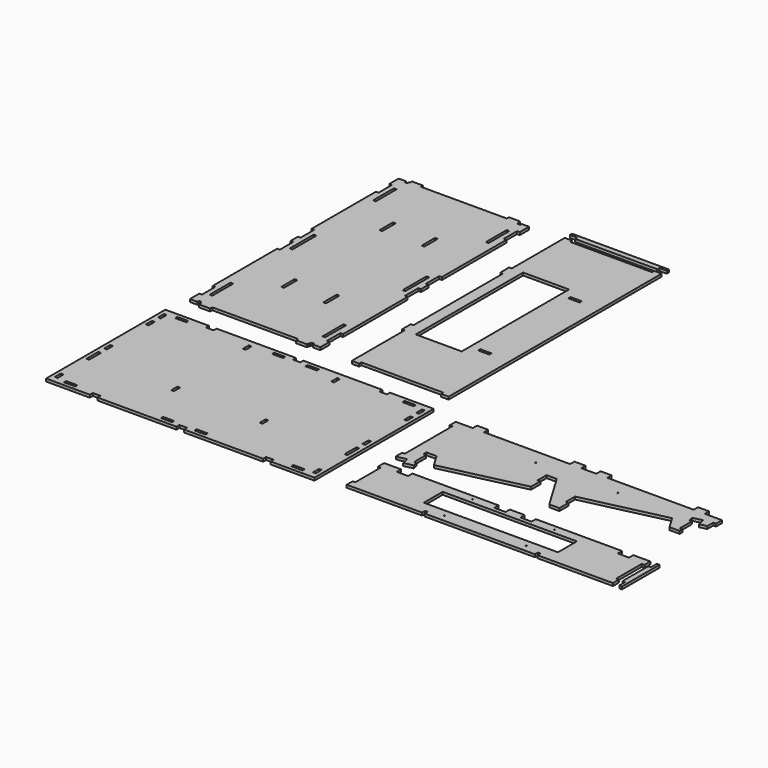
from build123d import *

# Parameters (mm, degrees)
F1_W     = 18.288
F1_H     = 177.8
F1_H_2   = 114.3
F1_H_3   = 203.2
F1_W_2   = 76.2
F1_H_4   = 18.288
F2_DEPTH = 18.288
F1_W_3   = 50.8
F1_H_5   = 76.2
F1_W_4   = 558.8
F1_H_6   = 50.8
F1_R     = 3.4925
F1_H_7   = 36.576
F1_H_8   = 25.4
F1_W_5   = 914.4
F1_H_9   = 161.1005576621
F1_H_10  = 217.424


# Not quite as in the source:
# - a variable given as a bare number and used for a length is read in inches; the dataset says mm whatever the document's units were


with BuildPart() as f2:
    # F1 (on Top) → F2 (new body)
    with BuildSketch(Plane.XY):
        Polygon((-889, 764.9814906911), (-889, 685.8), (-838.2, 685.8), (-838.2, 698.5), (-819.912, 698.5), (-819.912, 685.8), (-812.8, 685.8), (-736.6, 685.8), (-152.4, 685.8), (-76.2, 685.8), (-69.088, 685.8), (-69.088, 698.5), (-50.8, 698.5), (-50.8, 685.8), (0, 685.8), (0, 764.9814906911), (-18.288, 764.9814906911), (-18.288, 879.2814906911), (0, 879.2814906911), (0, 1428.75), (-18.288, 1428.75), (-18.288, 1543.05), (0, 1543.05), (0, 1606.55), (-18.288, 1606.55), (-18.288, 1720.85), (0, 1720.85), (0, 2270.3185093089), (-18.288, 2270.3185093089), (-18.288, 2384.6185093089), (0, 2384.6185093089), (0, 2463.8), (-50.8, 2463.8), (-50.8, 2451.1), (-69.088, 2451.1), (-69.088, 2463.8), (-76.2, 2463.8), (-152.4, 2463.8), (-736.6, 2463.8), (-812.8, 2463.8), (-819.912, 2463.8), (-819.912, 2451.1), (-838.2, 2451.1), (-838.2, 2463.8), (-889, 2463.8), (-889, 2384.6185093089), (-870.712, 2384.6185093089), (-870.712, 2270.3185093089), (-889, 2270.3185093089), (-889, 1720.85), (-870.712, 1720.85), (-870.712, 1606.55), (-889, 1606.55), (-889, 1543.05), (-870.712, 1543.05), (-870.712, 1428.75), (-889, 1428.75), (-889, 879.2814906911), (-870.712, 879.2814906911), (-870.712, 764.9814906911), align=None)
        with Locations((-829.056, 878.8908)):
            Rectangle(F1_W, F1_H, mode=Mode.SUBTRACT)
        with Locations((-59.944, 878.8908)):
            Rectangle(F1_W, F1_H, mode=Mode.SUBTRACT)
        with Locations((-587.756, 1155.7)):
            Rectangle(F1_W, F1_H_2, mode=Mode.SUBTRACT)
        with Locations((-301.244, 1155.7)):
            Rectangle(F1_W, F1_H_2, mode=Mode.SUBTRACT)
        with Locations((-829.056, 1574.8)):
            Rectangle(F1_W, F1_H_3, mode=Mode.SUBTRACT)
        with Locations((-59.944, 1574.8)):
            Rectangle(F1_W, F1_H_3, mode=Mode.SUBTRACT)
        with Locations((-587.756, 1993.9)):
            Rectangle(F1_W, F1_H_2, mode=Mode.SUBTRACT)
        with Locations((-301.244, 1993.9)):
            Rectangle(F1_W, F1_H_2, mode=Mode.SUBTRACT)
        with Locations((-829.056, 2270.7092)):
            Rectangle(F1_W, F1_H, mode=Mode.SUBTRACT)
        with Locations((-59.944, 2270.7092)):
            Rectangle(F1_W, F1_H, mode=Mode.SUBTRACT)
        with Locations((-774.7, 2472.944)):
            Rectangle(F1_W_2, F1_H_4)
        with Locations((-114.3, 2472.944)):
            Rectangle(F1_W_2, F1_H_4)
        with Locations((-114.3, 676.656)):
            Rectangle(F1_W_2, F1_H_4)
        with Locations((-774.7, 676.656)):
            Rectangle(F1_W_2, F1_H_4)
    extrude(amount=F2_DEPTH)


with BuildPart() as f2b:
    # F1 (on Top) → F2, piece 2 (new body)
    with BuildSketch(Plane.XY):
        Polygon((228.6, 1117.6), (228.6, 685.8), (279.4, 685.8), (838.2, 685.8), (889, 685.8), (889, 2463.8), (838.2, 2463.8), (279.4, 2463.8), (228.6, 2463.8), (228.6, 2032), (228.6, 1955.8), (228.6, 1193.8), align=None)
        with Locations((716.788, 1190.244)):
            Rectangle(F1_W_2, F1_H_4, mode=Mode.SUBTRACT)
        Polygon((304.8, 1574.8), (304.8, 2032), (617.6190740756, 2032), (617.6190740756, 1574.8), (617.6190740756, 1117.6), (304.8, 1117.6), align=None, mode=Mode.SUBTRACT)
        with Locations((716.788, 1959.356)):
            Rectangle(F1_W_2, F1_H_4, mode=Mode.SUBTRACT)
        with Locations((254, 676.656)):
            Rectangle(F1_W_3, F1_H_4)
        with Locations((863.6, 676.656)):
            Rectangle(F1_W_3, F1_H_4)
        with Locations((219.456, 1155.7)):
            Rectangle(F1_W, F1_H_5)
        with Locations((219.456, 1993.9)):
            Rectangle(F1_W, F1_H_5)
        with Locations((254, 2472.944)):
            Rectangle(F1_W_3, F1_H_4)
        with Locations((863.6, 2472.944)):
            Rectangle(F1_W_3, F1_H_4)
    extrude(amount=F2_DEPTH)


with BuildPart() as f2c:
    # F1 (on Top) → F2, piece 3 (new body)
    with BuildSketch(Plane.XY):
        Polygon((228.6, 2525.776), (279.4, 2525.776), (838.2, 2525.776), (889, 2525.776), (889, 2544.064), (228.6, 2544.064), align=None)
        with Locations((558.8, 2516.632)):
            Rectangle(F1_W_4, F1_H_4)
    extrude(amount=F2_DEPTH)


with BuildPart() as f2d:
    # F1 (on Top) → F2, piece 4 (new body)
    with BuildSketch(Plane.XY):
        Polygon((914.4, -508), (914.4, 508), (615.95, 508), (615.95, 482.6), (565.15, 482.6), (565.15, 508), (25.4, 508), (25.4, 482.6), (-25.4, 482.6), (-25.4, 508), (-565.15, 508), (-565.15, 482.6), (-615.95, 482.6), (-615.95, 508), (-914.4, 508), (-914.4, -508), (-615.95, -508), (-615.95, -482.6), (-565.15, -482.6), (-565.15, -508), (-25.4, -508), (-25.4, -482.6), (25.4, -482.6), (25.4, -508), (565.15, -508), (565.15, -482.6), (615.95, -482.6), (615.95, -508), align=None)
        with Locations((-879.856, -438.912)):
            Rectangle(F1_W, F1_H_6, mode=Mode.SUBTRACT)
        with Locations((-774.7, -473.456)):
            Rectangle(F1_W_2, F1_H_4, mode=Mode.SUBTRACT)
        Polygon((-889, -196.088), (-889, -145.288), (-889, -94.488), (-870.712, -94.488), (-870.712, -145.288), (-870.712, -196.088), align=None, mode=Mode.SUBTRACT)
        with Locations((-114.3, -473.456)):
            Rectangle(F1_W_2, F1_H_4, mode=Mode.SUBTRACT)
        with Locations((-301.244, -170.688)):
            Rectangle(F1_W, F1_H_6, mode=Mode.SUBTRACT)
        with Locations((-879.856, -18.288)):
            Rectangle(F1_W, F1_H_6, mode=Mode.SUBTRACT)
        with Locations((114.3, -473.456)):
            Rectangle(F1_W_2, F1_H_4, mode=Mode.SUBTRACT)
        with Locations((301.244, -170.688)):
            Rectangle(F1_W, F1_H_6, mode=Mode.SUBTRACT)
        with Locations((774.7, -473.456)):
            Rectangle(F1_W_2, F1_H_4, mode=Mode.SUBTRACT)
        with Locations((879.856, -438.912)):
            Rectangle(F1_W, F1_H_6, mode=Mode.SUBTRACT)
        Polygon((870.712, -94.488), (889, -94.488), (889, -145.288), (889, -196.088), (870.712, -196.088), (870.712, -145.288), align=None, mode=Mode.SUBTRACT)
        with Locations((879.856, -18.288)):
            Rectangle(F1_W, F1_H_6, mode=Mode.SUBTRACT)
        with Locations((-879.856, 337.312)):
            Rectangle(F1_W, F1_H_6, mode=Mode.SUBTRACT)
        with Locations((-879.856, 438.912)):
            Rectangle(F1_W, F1_H_6, mode=Mode.SUBTRACT)
        with Locations((-774.7, 473.456)):
            Rectangle(F1_W_2, F1_H_4, mode=Mode.SUBTRACT)
        with Locations((-301.244, 438.912)):
            Rectangle(F1_W, F1_H_6, mode=Mode.SUBTRACT)
        with Locations((-114.3, 473.456)):
            Rectangle(F1_W_2, F1_H_4, mode=Mode.SUBTRACT)
        with Locations((301.244, 438.912)):
            Rectangle(F1_W, F1_H_6, mode=Mode.SUBTRACT)
        with Locations((114.3, 473.456)):
            Rectangle(F1_W_2, F1_H_4, mode=Mode.SUBTRACT)
        with Locations((879.856, 337.312)):
            Rectangle(F1_W, F1_H_6, mode=Mode.SUBTRACT)
        with Locations((879.856, 438.912)):
            Rectangle(F1_W, F1_H_6, mode=Mode.SUBTRACT)
        with Locations((774.7, 473.456)):
            Rectangle(F1_W_2, F1_H_4, mode=Mode.SUBTRACT)
    extrude(amount=F2_DEPTH)


with BuildPart() as f2e:
    # F1 (on Top) → F2, piece 5 (new body)
    with BuildSketch(Plane.XY):
        Polygon((1215.8314906911, 464.312), (1117.6, 464.312), (1117.6, 413.512), (1117.6, 7.112), (1117.6, -43.688), (1166.3086785572, -32.5545877583), (1215.8314906911, -21.235087842), (1215.8314906911, 66.548), (1197.5434906911, 66.548), (1197.5434906911, 91.948), (1215.8314906911, 91.948), (1266.6314906911, 91.948), (1320.2245772409, 2.6261890836), (1879.6, 130.4834285714), (1879.6, 210.312), (1861.312, 210.312), (1861.312, 286.512), (1879.6, 286.512), (1930.4, 286.512), (2006.6, 159.512), (2133.6, 188.5405714286), (2692.9754227591, 316.3978109164), (2797.3685093089, 340.259087842), (2793.2934893391, 358.0873002102), (2780.9127863056, 355.2574252311), (2773.8380988579, 386.2091828148), (2835.7416140252, 400.3585577102), (2846.8913214428, 351.5785877583), (2895.6, 362.712), (2895.6, 413.512), (2895.6, 464.312), (2797.3685093089, 464.312), (2721.1685093089, 464.312), (2133.6, 464.312), (2057.4, 464.312), (1955.8, 464.312), (1879.6, 464.312), (1292.0314906911, 464.312), align=None)
        with Locations((1727.2, 362.712)):
            Circle(F1_R, mode=Mode.SUBTRACT)
        with Locations((2286, 362.712)):
            Circle(F1_R, mode=Mode.SUBTRACT)
        with Locations((1253.9314906911, 482.6)):
            Rectangle(F1_W_2, F1_H_7)
        with Locations((1108.456, 438.912)):
            Rectangle(F1_W, F1_H_6)
        with Locations((1108.456, -18.288)):
            Rectangle(F1_W, F1_H_6)
        Polygon((1215.8314906911, -21.235087842), (1166.3086785572, -32.5545877583), (1177.4583859748, -81.3345577102), (1239.3619011421, -67.1851828148), (1232.2872136944, -36.2334252311), (1219.9065106609, -39.0633002102), align=None)
        Polygon((2133.6, 188.5405714286), (2006.6, 159.512), (2082.8, 32.512), (2133.6, 32.512), (2133.6, 108.712), align=None)
        with Locations((2142.744, 70.612)):
            Rectangle(F1_W, F1_H_5)
        with Locations((1917.7, 482.6)):
            Rectangle(F1_W_2, F1_H_7)
        with Locations((2095.5, 482.6)):
            Rectangle(F1_W_2, F1_H_7)
        with Locations((2759.2685093089, 482.6)):
            Rectangle(F1_W_2, F1_H_7)
        Polygon((2797.3685093089, 340.259087842), (2692.9754227591, 316.3978109164), (2746.5685093089, 227.076), (2797.3685093089, 227.076), (2797.3685093089, 252.476), align=None)
        with Locations((2806.5125093089, 239.776)):
            Rectangle(F1_W, F1_H_8)
        with Locations((2904.744, 438.912)):
            Rectangle(F1_W, F1_H_6)
    extrude(amount=F2_DEPTH)


with BuildPart() as f2f:
    # F1 (on Top) → F2, piece 6 (new body)
    with BuildSketch(Plane.XY):
        with Locations((1108.456, -170.688)):
            Rectangle(F1_W, F1_H_6)
        with Locations((1108.456, -438.912)):
            Rectangle(F1_W, F1_H_6)
        Polygon((1215.8314906911, -145.288), (1117.6, -145.288), (1117.6, -196.088), (1117.6, -413.512), (1117.6, -464.312), (1612.9, -464.312), (1612.9, -438.912), (1631.188, -438.912), (1631.188, -464.312), (2382.012, -464.312), (2382.012, -438.912), (2400.3, -438.912), (2400.3, -464.312), (2895.6, -464.312), (2895.6, -413.512), (2895.6, -196.088), (2895.6, -145.288), (2797.3685093089, -145.288), (2797.3685093089, -181.864), (2721.1685093089, -181.864), (2721.1685093089, -145.288), (2133.6, -145.288), (2133.6, -181.864), (2057.4, -181.864), (2057.4, -145.288), (1955.8, -145.288), (1955.8, -181.864), (1879.6, -181.864), (1879.6, -145.288), (1292.0314906911, -145.288), (1292.0314906911, -181.864), (1215.8314906911, -181.864), align=None)
        with Locations((1727.2, -417.1002788311)):
            Circle(F1_R, mode=Mode.SUBTRACT)
        with Locations((1727.2, -177.038)):
            Circle(F1_R, mode=Mode.SUBTRACT)
        with Locations((2286, -417.1002788311)):
            Circle(F1_R, mode=Mode.SUBTRACT)
        with Locations((2006.6, -289.3382788311)):
            Rectangle(F1_W_5, F1_H_9, mode=Mode.SUBTRACT)
        with Locations((2286, -177.038)):
            Circle(F1_R, mode=Mode.SUBTRACT)
        with Locations((2904.744, -438.912)):
            Rectangle(F1_W, F1_H_6)
        with Locations((2904.744, -170.688)):
            Rectangle(F1_W, F1_H_6)
    extrude(amount=F2_DEPTH)


with BuildPart() as f2g:
    # F1 (on Top) → F2, piece 7 (new body)
    with BuildSketch(Plane.XY):
        with Locations((2948.432, -304.8)):
            Rectangle(F1_W, F1_H_10)
        Polygon((2957.576, -145.288), (2957.576, -196.088), (2957.576, -413.512), (2957.576, -464.312), (2975.864, -464.312), (2975.864, -145.288), align=None)
    extrude(amount=F2_DEPTH)


solid = Compound([f2.part, f2b.part, f2c.part, f2d.part, f2e.part, f2f.part, f2g.part])
